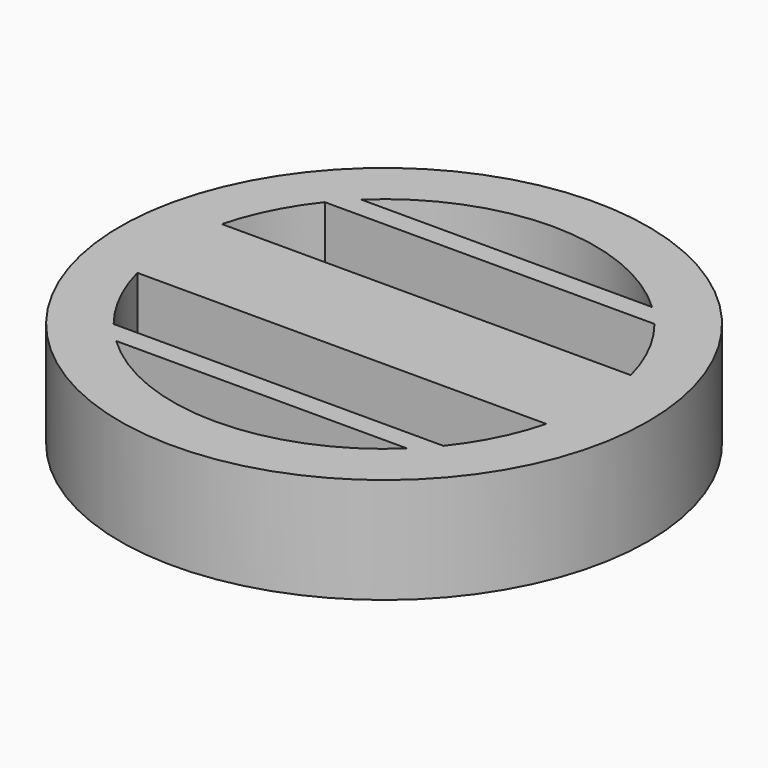
from build123d import *

# Parameters (mm, degrees)
F0_R     = 5
F1_DEPTH = 2
F2_DEPTH = 2
F3_DEPTH = 2
F4_DEPTH = 2


with BuildPart() as f1:
    # F0 (on Top) → F1 (new body)
    with BuildSketch(Plane.XY):
        Circle(F0_R)
        with BuildLine():
            ThreePointArc((3.8729833462, 1), (3.9681187851, 0.5040171699), (4, 0))
            ThreePointArc((4, 0), (3.9681187851, -0.5040171699), (3.8729833462, -1))
            ThreePointArc((3.8729833462, -1), (3.5772466103, -1.789778391), (3.1224989992, -2.5))
            ThreePointArc((3.1224989992, -2.5), (2.9455449899, -2.7062455011), (2.7549954628, -2.9))
            ThreePointArc((2.7549954628, -2.9), (0, -4), (-2.7549954628, -2.9))
            ThreePointArc((-2.7549954628, -2.9), (-2.9455449899, -2.7062455011), (-3.1224989992, -2.5))
            ThreePointArc((-3.1224989992, -2.5), (-3.5772466103, -1.789778391), (-3.8729833462, -1))
            ThreePointArc((-3.8729833462, -1), (-4, 0), (-3.8729833462, 1))
            ThreePointArc((-3.8729833462, 1), (-3.5772466103, 1.789778391), (-3.1224989992, 2.5))
            ThreePointArc((-3.1224989992, 2.5), (-2.9455449899, 2.7062455011), (-2.7549954628, 2.9))
            ThreePointArc((-2.7549954628, 2.9), (0, 4), (2.7549954628, 2.9))
            ThreePointArc((2.7549954628, 2.9), (2.9455449899, 2.7062455011), (3.1224989992, 2.5))
            ThreePointArc((3.1224989992, 2.5), (3.5772466103, 1.789778391), (3.8729833462, 1))
        make_face(mode=Mode.SUBTRACT)
    extrude(amount=F1_DEPTH)

    # F0 (on Top) → F2 (join)
    with BuildSketch(Plane.XY):
        with BuildLine():
            ThreePointArc((3.8729833462, -1), (3.9681187851, -0.5040171699), (4, 0))
            ThreePointArc((4, 0), (3.9681187851, 0.5040171699), (3.8729833462, 1))
            Line((3.8729833462, 1), (-2.1040285937, 1))
            Line((-2.1040285937, 1), (-3.8729833462, 1))
            ThreePointArc((-3.8729833462, 1), (-4, 0), (-3.8729833462, -1))
            Line((-3.8729833462, -1), (-2.1040285937, -1))
            Line((-2.1040285937, -1), (3.8729833462, -1))
        make_face()
    extrude(amount=F2_DEPTH)

    # F0 (on Top) → F3 (join)
    with BuildSketch(Plane.XY):
        with BuildLine():
            Line((-2.1040285937, 2.5), (3.1224989992, 2.5))
            ThreePointArc((3.1224989992, 2.5), (2.9455449899, 2.7062455011), (2.7549954628, 2.9))
            Line((2.7549954628, 2.9), (-0.8741539787, 2.9))
            Line((-0.8741539787, 2.9), (-2.7549954628, 2.9))
            ThreePointArc((-2.7549954628, 2.9), (-2.9455449899, 2.7062455011), (-3.1224989992, 2.5))
            Line((-3.1224989992, 2.5), (-2.1040285937, 2.5))
        make_face()
    extrude(amount=F3_DEPTH)

    # F0 (on Top) → F4 (join)
    with BuildSketch(Plane.XY):
        with BuildLine():
            ThreePointArc((2.7549954628, -2.9), (2.9455449899, -2.7062455011), (3.1224989992, -2.5))
            Line((3.1224989992, -2.5), (-2.1040285937, -2.5))
            Line((-2.1040285937, -2.5), (-3.1224989992, -2.5))
            ThreePointArc((-3.1224989992, -2.5), (-2.9455449899, -2.7062455011), (-2.7549954628, -2.9))
            Line((-2.7549954628, -2.9), (-1.2980791507, -2.9))
            Line((-1.2980791507, -2.9), (2.7549954628, -2.9))
        make_face()
    extrude(amount=F4_DEPTH)


solid = f1.part
